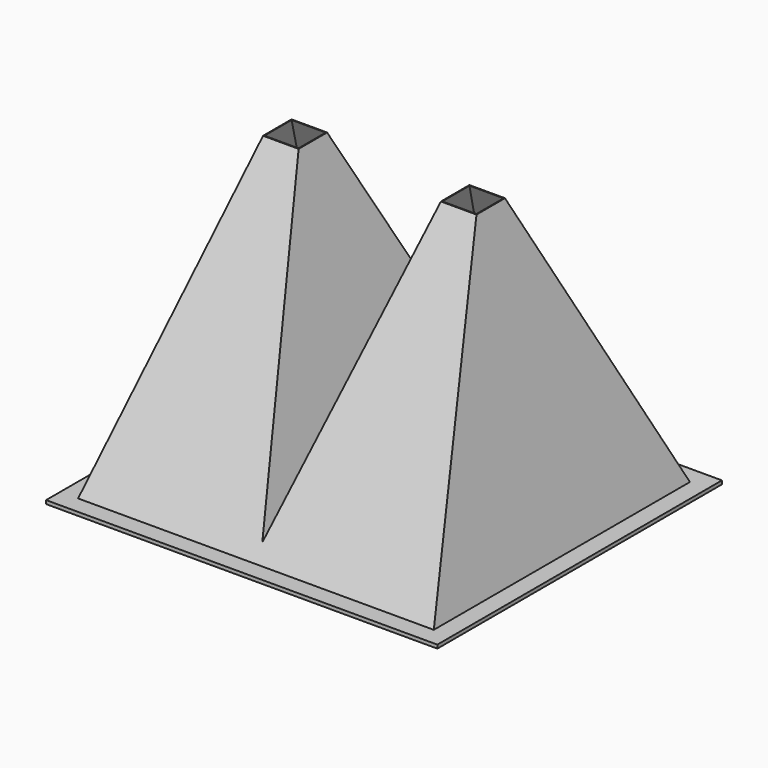
from build123d import *

# Parameters (mm, degrees)
F6_DEPTH      = 114.3
F6_DEPTH_BACK = 114.3
F8_DEPTH      = 127.001
F8_DEPTH_BACK = 127.001
F9_W          = 279.4
F9_H          = 254
F10_DEPTH     = 2.54
F11_T         = -0.508


# Not quite as in the source:
# - a pattern or mirror of a feature is missing from the dataset's text; its kind, count and spacing are read off the source's solid


with BuildPart() as f6:
    # F5 (on Front) → F6 (new body, two sides)
    with BuildSketch(Plane.XZ) as f6_sk:
        Polygon((-76.2, 203.2), (-127, 0), (127, 0), (76.2, 203.2), (50.8, 203.2), (0, 11.3592253257), (-50.8, 203.2), align=None)
    extrude(amount=F6_DEPTH)
    extrude(f6_sk.sketch, amount=-F6_DEPTH_BACK)

    # F7 (on Right) → F8 (cut, two sides)
    with BuildSketch(Plane.YZ) as f8_sk:
        Polygon((-114.3, 203.2), (-114.3, 0), (-12.7, 203.2), align=None)
    f8 = extrude(amount=-F8_DEPTH, mode=Mode.SUBTRACT) + extrude(f8_sk.sketch, amount=F8_DEPTH_BACK, mode=Mode.SUBTRACT)

    # F8_copies: F8 across plane
    add(f8.mirror(Plane.ZX), mode=Mode.SUBTRACT)

    # F9 (on face) → F10 (join)
    with BuildSketch(Plane(origin=(0, 0, 0), x_dir=(1, 0, 0), z_dir=(0, 0, -1))):
        Rectangle(F9_W, F9_H)
    extrude(amount=F10_DEPTH)

    # F11
    f11_openings = [f6.faces().sort_by_distance(p)[0] for p in [
        (0, 0, -2.54),
        (63.5, 0, 203.2),
        (-63.5, 0, 203.2),
    ]]
    offset(amount=F11_T, openings=f11_openings, kind=Kind.INTERSECTION)


solid = f6.part
